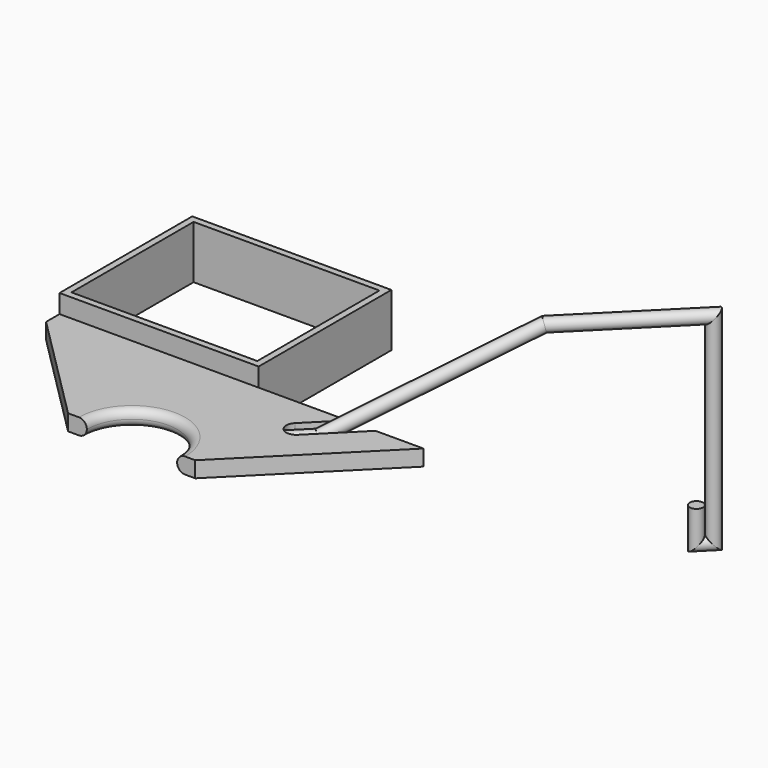
from build123d import *

# Parameters (mm, degrees)
F3_DEPTH      = 6
F3_DEPTH_BACK = 6
F4_R          = 5.99999
F5_W          = 150
F5_H          = 125
F5_W_2        = 140
F5_H_2        = 115
F6_DEPTH      = 20
F6_DEPTH_BACK = 20
F7_W          = 18.4257775545
F7_H          = 22.6281583309
F8_DEPTH      = 25
F8_DEPTH_BACK = 25
F12_R         = 5


# Not quite as in the source:
# - a fillet or chamfer is up to 0.001 mm smaller than in the source, because OpenCascade refuses the exact size
# - the program builds the solid bodies; features that only make, move or delete a surface that nothing else refers to are left out


with BuildPart() as f3:
    # F2 (on Top) → F3 (new body, two sides)
    with BuildSketch(Plane.XY) as f3_sk:
        with BuildLine():
            Line((-143.6767325086, 95.5261040182), (-48.1506284904, 0))
            Line((-48.1506284904, 0), (-34, 0))
            ThreePointArc((-34, 0), (0, 34), (34, 0))
            Line((34, 0), (47.630082774, 0))
            Line((47.630082774, 0), (143.1561867922, 95.5261040182))
            Line((143.1561867922, 95.5261040182), (107.040643459, 95.5261040182))
            Line((107.040643459, 95.5261040182), (74.4780500334, 62.9635105926))
            ThreePointArc((74.4780500334, 62.9635105926), (63.8714483156, 62.9635105926), (63.8714483156, 73.5701123104))
            Line((63.8714483156, 73.5701123104), (85.8274400234, 95.5261040182))
            Line((85.8274400234, 95.5261040182), (-143.6767325086, 95.5261040182))
        make_face()
    extrude(amount=F3_DEPTH)
    extrude(f3_sk.sketch, amount=-F3_DEPTH_BACK)

    # F4 (radius 6 in the source; OpenCascade refuses exactly that, so slightly less here)
    f4_edges = [f3.edges().sort_by_distance(p)[0] for p in [
        (0, 34, 6),
        (0, 34, -6),
    ]]
    fillet(f4_edges, radius=F4_R)

    # F5 (on Top) → F6 (join, two sides)
    with BuildSketch(Plane.XY) as f6_sk:
        with Locations((-56.0159248962, 158.0261040182)):
            Rectangle(F5_W, F5_H)
        with Locations((-56.0159248962, 158.0261040182)):
            Rectangle(F5_W_2, F5_H_2, mode=Mode.SUBTRACT)
    extrude(amount=F6_DEPTH)
    extrude(f6_sk.sketch, amount=-F6_DEPTH_BACK)

    # F7 (on Top) → F8 (cut, two sides)
    with BuildSketch(Plane.XY) as f8_sk:
        with Locations((-140.2288136734, 86.2188637257)):
            Rectangle(F7_W, F7_H)
    extrude(amount=F8_DEPTH, mode=Mode.SUBTRACT)
    extrude(f8_sk.sketch, amount=-F8_DEPTH_BACK, mode=Mode.SUBTRACT)


with BuildPart() as f13:
    # F13: sweep along a path in F10
    with BuildLine(Plane(origin=(0.4539688615, -0.4539688615, 0), x_dir=(0.7071067812, 0.7071067812, 0), z_dir=(0.7071067812, -0.7071067812, 0))) as f13_path:
        Line((333.9798068309, -57.8993414214), (333.9798068309, -82.8993414214))
        Line((333.9798068309, -82.8993414214), (343.9798068309, -82.8993414214))
        Line((343.9798068309, -82.8993414214), (343.9798068309, 67.1006585786))
        Line((343.9798068309, 67.1006585786), (243.9798068309, 67.1006585786))
        Line((243.9798068309, 67.1006585786), (109.8250394228, 0))
        Line((109.8250394228, 0), (88.6497050524, 0))
        Line((88.6497050524, 0), (38.6362485588, 0))
    # F12 (on plane+point) → F13 (sweep)
    with BuildSketch(Plane.XY.offset(-57.8993414214)):
        with Locations((236.7622852325, 235.4874759912)):
            Circle(F12_R)
    sweep(path=f13_path.line, transition=Transition.RIGHT)


solid = Compound([f3.part, f13.part])
